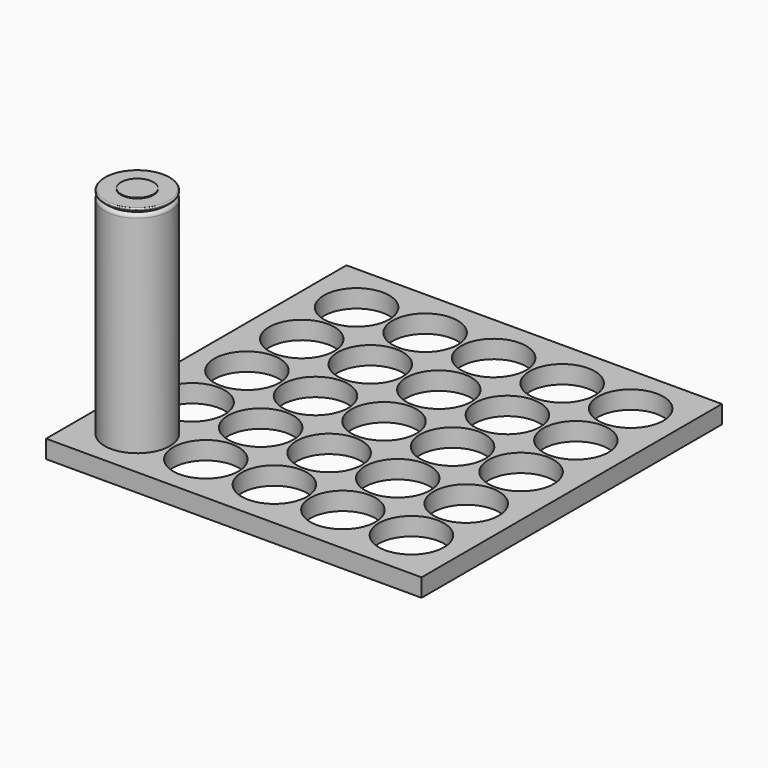
from build123d import *

# Parameters (mm, degrees)
F2_R     = 0.99999
F3_R     = 0.3017766953
F4_W     = 104.1
F4_H     = 104.1
F4_R     = 9.05
F5_DEPTH = 5


# Not quite as in the source:
# - a fillet or chamfer is up to 0.001 mm smaller than in the source, because OpenCascade refuses the exact size


with BuildPart() as f1:
    # F0 (on Front) → F1 (revolve)
    with BuildSketch(Plane.XZ):
        Polygon((0, 65), (0, 0), (9.05, 0), (9.05, 63.3736730193), (8.05, 63.3736730193), (8.05, 63.8736730193), (9.05, 64.05), (9.05, 64.8), (4.5, 64.8), (4.5, 65), align=None)
    revolve(axis=Axis((0, 0, 32.5), (0, 0, -1)))

    # F2 (radius 1 in the source; OpenCascade refuses exactly that, so slightly less here)
    f2_edges = [f1.edges().sort_by_distance(p)[0] for p in [
        (-9.05, 0, 0),
        (-9.05, 0, 63.373673),
    ]]
    fillet(f2_edges, radius=F2_R)

    # F3
    f3_edges = [f1.edges().sort_by_distance(p)[0] for p in [
        (-9.05, 0, 64.05),
        (-9.05, 0, 64.8),
    ]]
    fillet(f3_edges, radius=F3_R)


with BuildPart() as f5:
    # F4 (on Top) → F5 (new body)
    with BuildSketch(Plane.XY):
        with Locations((38, 38)):
            Rectangle(F4_W, F4_H)
        Circle(F4_R, mode=Mode.SUBTRACT)
        with Locations((19, 0)):
            Circle(F4_R, mode=Mode.SUBTRACT)
        with Locations((0, 19)):
            Circle(F4_R, mode=Mode.SUBTRACT)
        with Locations((19, 19)):
            Circle(F4_R, mode=Mode.SUBTRACT)
        with Locations((38, 0)):
            Circle(F4_R, mode=Mode.SUBTRACT)
        with Locations((57, 0)):
            Circle(F4_R, mode=Mode.SUBTRACT)
        with Locations((76, 0)):
            Circle(F4_R, mode=Mode.SUBTRACT)
        with Locations((38, 19)):
            Circle(F4_R, mode=Mode.SUBTRACT)
        with Locations((57, 19)):
            Circle(F4_R, mode=Mode.SUBTRACT)
        with Locations((76, 19)):
            Circle(F4_R, mode=Mode.SUBTRACT)
        with Locations((0, 38)):
            Circle(F4_R, mode=Mode.SUBTRACT)
        with Locations((0, 57)):
            Circle(F4_R, mode=Mode.SUBTRACT)
        with Locations((19, 38)):
            Circle(F4_R, mode=Mode.SUBTRACT)
        with Locations((19, 57)):
            Circle(F4_R, mode=Mode.SUBTRACT)
        with Locations((0, 76)):
            Circle(F4_R, mode=Mode.SUBTRACT)
        with Locations((19, 76)):
            Circle(F4_R, mode=Mode.SUBTRACT)
        with Locations((38, 38)):
            Circle(F4_R, mode=Mode.SUBTRACT)
        with Locations((57, 38)):
            Circle(F4_R, mode=Mode.SUBTRACT)
        with Locations((38, 57)):
            Circle(F4_R, mode=Mode.SUBTRACT)
        with Locations((57, 57)):
            Circle(F4_R, mode=Mode.SUBTRACT)
        with Locations((76, 38)):
            Circle(F4_R, mode=Mode.SUBTRACT)
        with Locations((76, 57)):
            Circle(F4_R, mode=Mode.SUBTRACT)
        with Locations((38, 76)):
            Circle(F4_R, mode=Mode.SUBTRACT)
        with Locations((57, 76)):
            Circle(F4_R, mode=Mode.SUBTRACT)
        with Locations((76, 76)):
            Circle(F4_R, mode=Mode.SUBTRACT)
    extrude(amount=F5_DEPTH)


solid = Compound([f1.part, f5.part])
